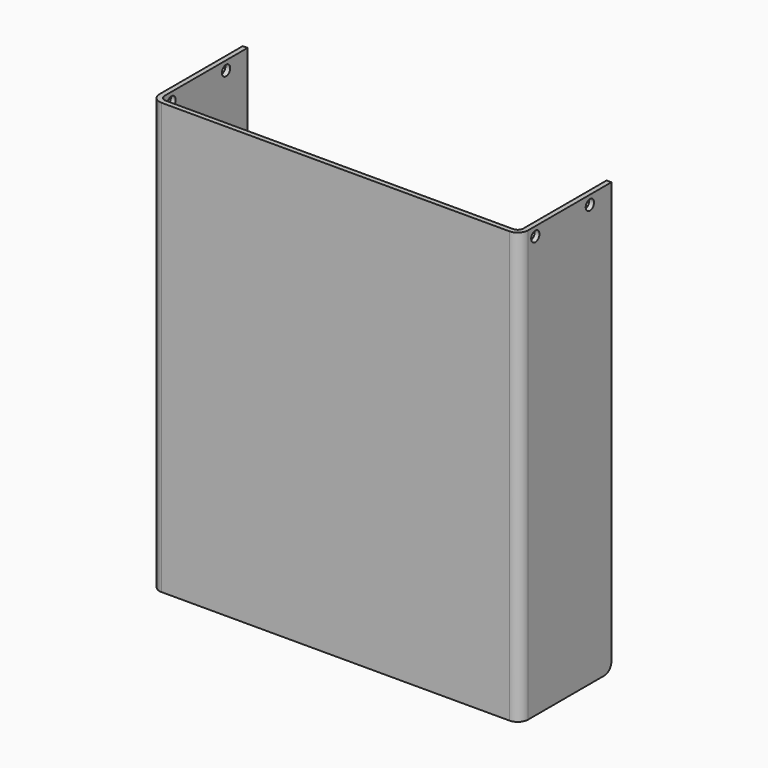
from build123d import *

# Parameters (mm, degrees)
F1_DEPTH = 152.4
F2_R     = 1.98374
F3_R     = 3.69316
F4_R     = 1.8288
F5_DEPTH = 130.41884
F6_R     = 3.175


with BuildPart() as f1:
    # F0 (on Top) → F1 (new body)
    with BuildSketch(Plane.XY):
        Polygon((0, 38.8047992), (0, 0), (-127, 0), (-127, 38.8047992), (-128.70942, 38.8047992), (-128.70942, -1.70942), (1.70942, -1.70942), (1.70942, 38.8047992), align=None)
    extrude(amount=F1_DEPTH)

    # F2
    f2_edges = [f1.edges().sort_by_distance(p)[0] for p in [
        (0, 0, 76.2),
        (-127, 0, 76.2),
    ]]
    fillet(f2_edges, radius=F2_R)

    # F3
    f3_edges = [f1.edges().sort_by_distance(p)[0] for p in [
        (1.70942, -1.70942, 76.2),
        (-128.70942, -1.70942, 76.2),
    ]]
    fillet(f3_edges, radius=F3_R)

    # F4 (on face) → F5 (cut, through all)
    with BuildSketch(Plane(origin=(-128.70942, 0, 0), x_dir=(0, -1, 0), z_dir=(-1, 0, 0))):
        with Locations((-29.2797992, 149.225)):
            Circle(F4_R)
        with Locations((-5.15874, 149.225)):
            Circle(F4_R)
    extrude(amount=-F5_DEPTH, mode=Mode.SUBTRACT)

    # F6
    f6_edges = [f1.edges().sort_by_distance(p)[0] for p in [
        (0.85471, 38.804799, 0),
        (-127.85471, 38.804799, 0),
    ]]
    fillet(f6_edges, radius=F6_R)


solid = f1.part
